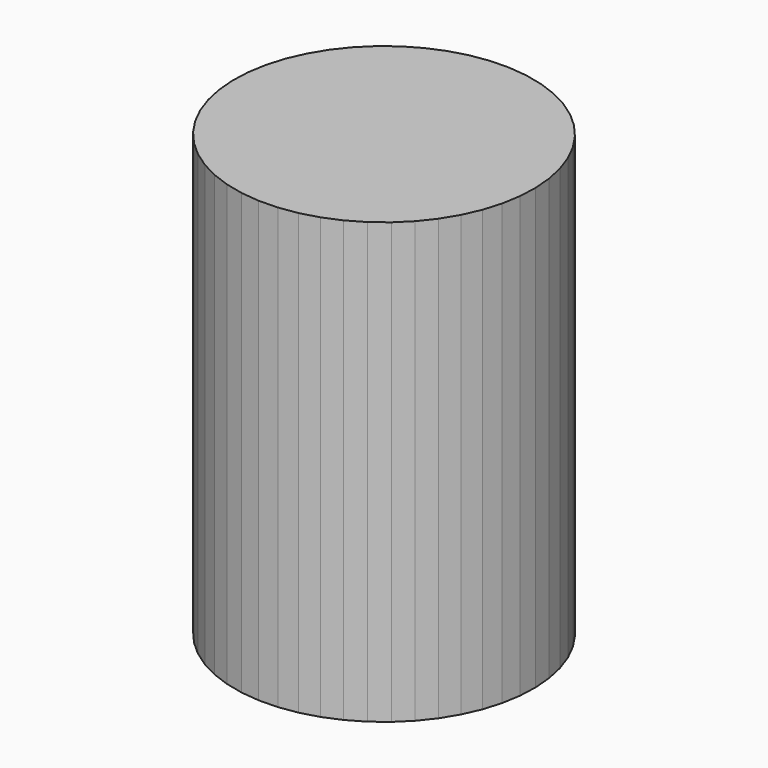
from build123d import *

# Parameters (mm, degrees)
F1_DEPTH = 25.4
F2_T     = -2.54


with BuildPart() as f1:
    # F0 (on Top) → F1 (new body)
    with BuildSketch(Plane.XY):
        Polygon((-7.453287064, -4.3146827775), (-6.853742525, -5.2148047835), (-6.1461103721, -6.0326862028), (-5.3415503872, -6.755428557), (-4.4527509618, -7.3716337674), (-3.4937289938, -7.8715839096), (-2.4796088325, -8.2473944714), (-1.4263837586, -8.4931386955), (-0.3506637608, -8.6049410489), (0.7305864139, -8.5810383416), (1.8003148046, -8.4218075336), (2.8416511552, -8.1297597898), (3.8381729697, -7.7095008777), (4.7741645036, -7.1676585313), (5.6348646113, -6.5127779281), (6.406699538, -5.7551869264), (7.0774969858, -4.906833189), (7.6366780783, -3.9810957609), (8.0754241955, -2.9925740745), (8.3868160491, -1.9568577072), (8.5659428036, -0.890280525), (8.6099795231, 0.190336913), (8.5182317221, 1.2679526241), (8.2921463183, 2.3255719649), (7.9352888136, 3.3465156466), (7.453287064, 4.3146827775), (6.853742525, 5.2148047835), (6.1461103721, 6.0326862028), (5.3415503872, 6.755428557), (4.4527509618, 7.3716337674), (3.4937289938, 7.8715839096), (2.4796088325, 8.2473944714), (1.4263837586, 8.4931386955), (0.3506637608, 8.6049410489), (-0.7305864139, 8.5810383416), (-1.8003148046, 8.4218075336), (-2.8416511552, 8.1297597898), (-3.8381729697, 7.7095008777), (-4.7741645036, 7.1676585313), (-5.6348646113, 6.5127779281), (-6.406699538, 5.7551869264), (-7.0774969858, 4.906833189), (-7.6366780783, 3.9810957609), (-8.0754241955, 2.9925740745), (-8.3868160491, 1.9568577072), (-8.5659428036, 0.890280525), (-8.6099795231, -0.190336913), (-8.5182317221, -1.2679526241), (-8.2921463183, -2.3255719649), (-7.9352888136, -3.3465156466), align=None)
    extrude(amount=F1_DEPTH)

    # F2
    f2_openings = [f1.faces().sort_by_distance(p)[0] for p in [
        (0, 0, 0),
    ]]
    offset(amount=F2_T, openings=f2_openings)


with BuildPart() as f1_1:
    # F3: moved
    add(f1.part.moved(Location((0, 0, -25.4))))


solid = f1_1.part
